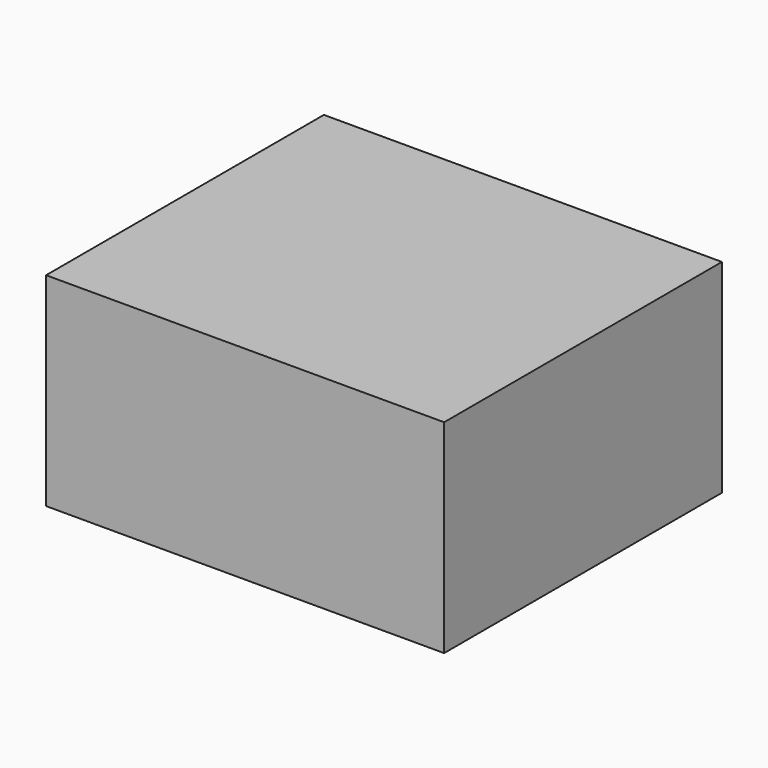
from build123d import *

# Parameters (mm, degrees)
F0_W     = 149.225
F0_H     = 76.2
F0_W_2   = 47.625
F0_H_2   = 34.925
F0_W_3   = 31.75
F0_H_3   = 19.05
F0_H_4   = 25.4
F0_H_5   = 31.75
F0_W_4   = 50.8
F1_DEPTH = 127
F2_W     = 149.225
F2_H     = 76.2
F3_DEPTH = 3.175


# Not quite as in the source:
# - a length typed as a fraction of an inch, garbled in the dataset ("3 / 203.2 mm" for 3/8 in), is restored


with BuildPart() as f1:
    # F0 (on Front) → F1 (new body)
    with BuildSketch(Plane.XZ):
        with Locations((-19.0595093454, -28.2635252237)):
            Rectangle(F0_W, F0_H)
        with Locations((-68.2720093454, -45.7260252237)):
            Rectangle(F0_W_2, F0_H_2, mode=Mode.SUBTRACT)
        with Locations((-19.2011359204, -31.6498865128)):
            Rectangle(F0_W_3, F0_H_3, mode=Mode.SUBTRACT)
        with Locations((-19.0595093454, -53.6635252237)):
            Rectangle(F0_W_2, F0_H_3, mode=Mode.SUBTRACT)
        with Locations((30.1529906546, -50.4885252237)):
            Rectangle(F0_W_2, F0_H_4, mode=Mode.SUBTRACT)
        with Locations((-76.2095093454, -9.2135252237)):
            Rectangle(F0_W_3, F0_H_5, mode=Mode.SUBTRACT)
        with Locations((-25.4095093454, -6.0385252237)):
            Rectangle(F0_W_4, F0_H_4, mode=Mode.SUBTRACT)
        with Locations((28.5654906546, -6.0385252237)):
            Rectangle(F0_W_4, F0_H_4, mode=Mode.SUBTRACT)
    extrude(amount=F1_DEPTH)

    # F2 (on face) → F3 (join)
    with BuildSketch(Plane.XZ.offset(127)):
        with Locations((-19.0595093454, -28.2635252237)):
            Rectangle(F2_W, F2_H)
    extrude(amount=F3_DEPTH)


solid = f1.part
